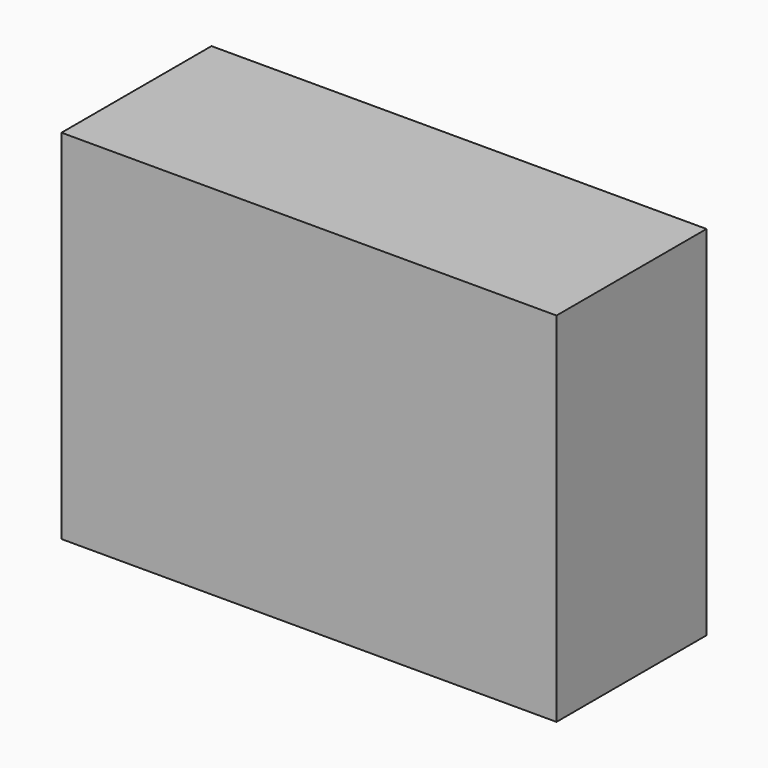
from build123d import *

# Parameters (mm, degrees)
F0_W     = 67.0537650585
F0_H     = 48.4633408487
F1_DEPTH = 25.4


# Not quite as in the source:
# - the program builds the solid bodies; features that only make, move or delete a surface that nothing else refers to are left out


with BuildPart() as f1:
    # F0 (on Front) → F1 (new body)
    with BuildSketch(Plane.XZ):
        with Locations((-10.5370208621, 39.106303826)):
            Rectangle(F0_W, F0_H)
    extrude(amount=F1_DEPTH)


solid = f1.part
